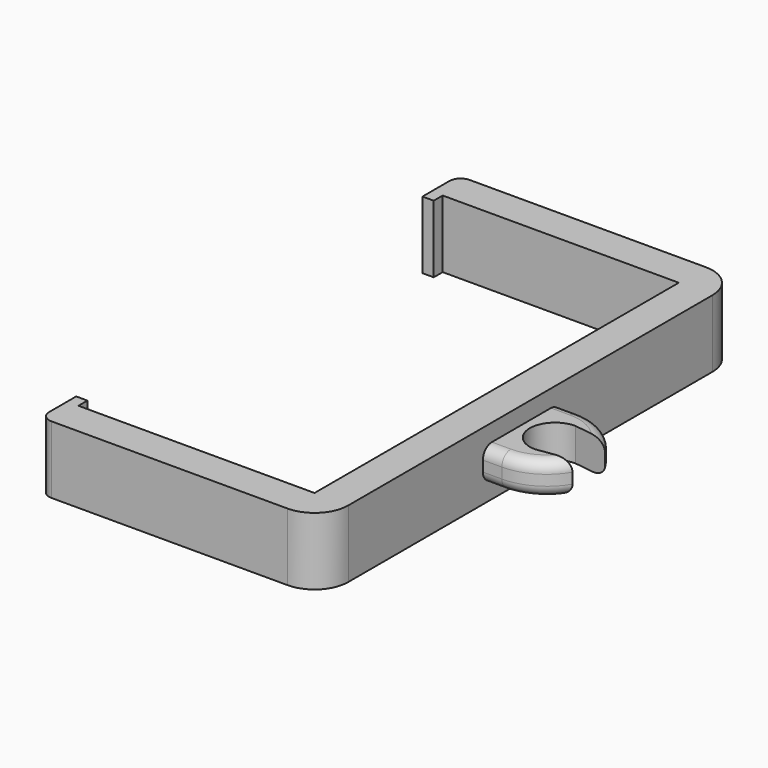
from build123d import *

# Parameters (mm, degrees)
F1_DEPTH    = 6
F2_W        = 8.5644074716
F2_H        = 2.9347334579
F3_DEPTH    = 6
F5_DEPTH    = 25
F6_T1_DEPTH = 24.4869357348
F6_T3_DEPTH = 24.4827319302
F7_R        = 3
F8_R        = 1


# Not quite as in the source:
# - a fillet or chamfer that OpenCascade refuses, or shapes differently, is made with other operations: its cross-section is extruded or revolved along the edge and cut away or added


with BuildPart() as f1:
    # F0 (on Top) → F1 (new body)
    with BuildSketch(Plane.XY):
        Polygon((-4.42252215, 28.2665032521), (16.57747785, 28.2665032521), (16.57747785, -12.2334967479), (-4.42252215, -12.2334967479), (-4.42252215, -11.2334967479), (-5.42252215, -11.2334967479), (-5.42252215, -13.2334967479), (-5.42252215, -15.2334967479), (-4.42252215, -15.2334967479), (16.57747785, -15.2334967479), (19.57747785, -15.2334967479), (19.57747785, -13.2334967479), (19.57747785, 27.2665032521), (19.57747785, 31.2665032521), (16.57747785, 31.2665032521), (-4.42252215, 31.2665032521), (-5.42252215, 31.2665032521), (-5.42252215, 27.2665032521), (-4.42252215, 27.2665032521), align=None)
    extrude(amount=F1_DEPTH)

    # F2 (on face) → F3 (join)
    with BuildSketch(Plane.YZ.offset(19.57747785)):
        with Locations((7.0165032521, 3)):
            Rectangle(F2_W, F2_H)
    extrude(amount=F3_DEPTH)

    # F4 (on face) → F5 (cut)
    with BuildSketch(Plane.XY.offset(4.4673667289)):
        with BuildLine():
            Line((25.57747785, 8.833928965), (22.57747785, 9.2672181241))
            ThreePointArc((22.57747785, 9.2672181241), (20.32747785, 7.0172181241), (22.57747785, 4.7672181241))
            Line((22.57747785, 4.7672181241), (25.57747785, 5.2005072832))
            Line((25.57747785, 5.2005072832), (25.57747785, 8.833928965))
        make_face()
    extrude(amount=-F5_DEPTH, mode=Mode.SUBTRACT)

    # F6: fillet of radius 5 on 2 edges, made by hand

    # F6_s2 → F6_t1 (cut)
    with BuildSketch(Plane.XY.offset(-9.2434678674)):
        with BuildLine():
            ThreePointArc((21.2670373946, 2.7342995163), (23.7500837932, 3.3944284833), (25.57747785, 5.2005072832))
            Line((25.57747785, 5.2005072832), (25.57747785, 2.7342995163))
            Line((25.57747785, 2.7342995163), (21.2670373946, 2.7342995163))
        make_face()
    extrude(amount=F6_T1_DEPTH, mode=Mode.SUBTRACT)

    # F6_s4 → F6_t3 (cut)
    with BuildSketch(Plane.XY.offset(-9.2413659651)):
        with BuildLine():
            ThreePointArc((21.2678781556, 11.2987069879), (23.7502046967, 10.6389898062), (25.57747785, 8.833928965))
            Line((25.57747785, 8.833928965), (25.57747785, 11.2987069879))
            Line((25.57747785, 11.2987069879), (21.2678781556, 11.2987069879))
        make_face()
    extrude(amount=F6_T3_DEPTH, mode=Mode.SUBTRACT)

    # F7
    f7_edges = [f1.edges().sort_by_distance(p)[0] for p in [
        (19.577478, -15.233497, 3),
        (19.577478, 31.266503, 3),
    ]]
    fillet(f7_edges, radius=F7_R)

    # F8
    f8_edges = [f1.edges().sort_by_distance(p)[0] for p in [
        (-5.422522, -15.233497, 3),
        (-5.422522, 31.266503, 3),
        (23.750084, 3.394428, 4.467367),
        (23.750084, 3.394428, 1.532633),
        (23.750205, 10.63899, 1.532633),
        (23.750205, 10.63899, 4.467367),
        (20.422678, 11.298707, 1.532633),
        (20.422258, 2.7343, 1.532633),
        (20.422258, 2.7343, 4.467367),
        (20.422678, 11.298707, 4.467367),
    ]]
    fillet(f8_edges, radius=F8_R)


solid = f1.part
